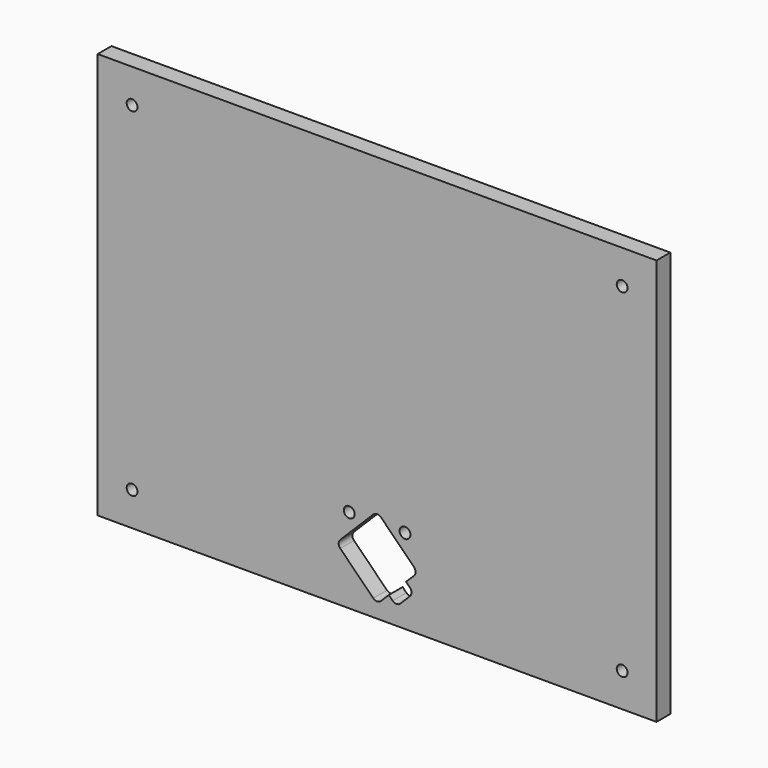
from build123d import *

# Parameters (mm, degrees)
F0_W     = 412.7
F0_H     = 300
F0_R     = 4
F1_DEPTH = 12.7


# Not quite as in the source:
# - ends of sketch curves that miss each other by under 0.0002 mm in the source are joined
# - a length typed as a fraction of an inch, garbled in the dataset ("3 / 203.2 mm" for 3/8 in), is restored


with BuildPart() as f1:
    # F0 (on Front) → F1 (new body)
    with BuildSketch(Plane.XZ):
        Rectangle(F0_W, F0_H)
        with Locations((-180.95, -125)):
            Circle(F0_R, mode=Mode.SUBTRACT)
        with BuildLine():
            ThreePointArc((-27.2236111247, -113.1947061247), (-28.395184, -110.366279), (-27.2236111247, -107.5378518753))
            Line((-27.2236111247, -107.5378518753), (-2.828427, -83.142668))
            ThreePointArc((-2.828427, -83.142668), (0, -81.971095), (2.8284271247, -83.1426678753))
            Line((2.8284271247, -83.1426678753), (27.223611, -107.537852))
            ThreePointArc((27.223611, -107.537852), (28.395184, -110.366279), (27.2236111247, -113.1947061247))
            Line((27.2236111247, -113.1947061247), (21.38998, -119.028337))
            Line((21.38998, -119.028337), (24.218407, -121.856764))
            ThreePointArc((24.218407, -121.856764), (25.38998, -124.685191), (24.2184071247, -127.5136181247))
            Line((24.2184071247, -127.5136181247), (17.147339, -134.584686))
            ThreePointArc((17.147339, -134.584686), (14.318912, -135.756259), (11.4904848753, -134.5846861247))
            Line((11.4904848753, -134.5846861247), (8.662058, -131.756259))
            Line((8.662058, -131.756259), (2.828427, -137.58989))
            ThreePointArc((2.828427, -137.58989), (0, -138.761463), (-2.8284271247, -137.5898901247))
            Line((-2.8284271247, -137.5898901247), (-27.2236111247, -113.1947061247))
        make_face(mode=Mode.SUBTRACT)
        with Locations((-20.590066, -87.466386)):
            Circle(F0_R, mode=Mode.SUBTRACT)
        with Locations((20.590066, -87.466386)):
            Circle(F0_R, mode=Mode.SUBTRACT)
        with Locations((180.95, -125)):
            Circle(F0_R, mode=Mode.SUBTRACT)
        with Locations((-180.95, 125)):
            Circle(F0_R, mode=Mode.SUBTRACT)
        with Locations((180.95, 125)):
            Circle(F0_R, mode=Mode.SUBTRACT)
    extrude(amount=F1_DEPTH)


solid = f1.part
